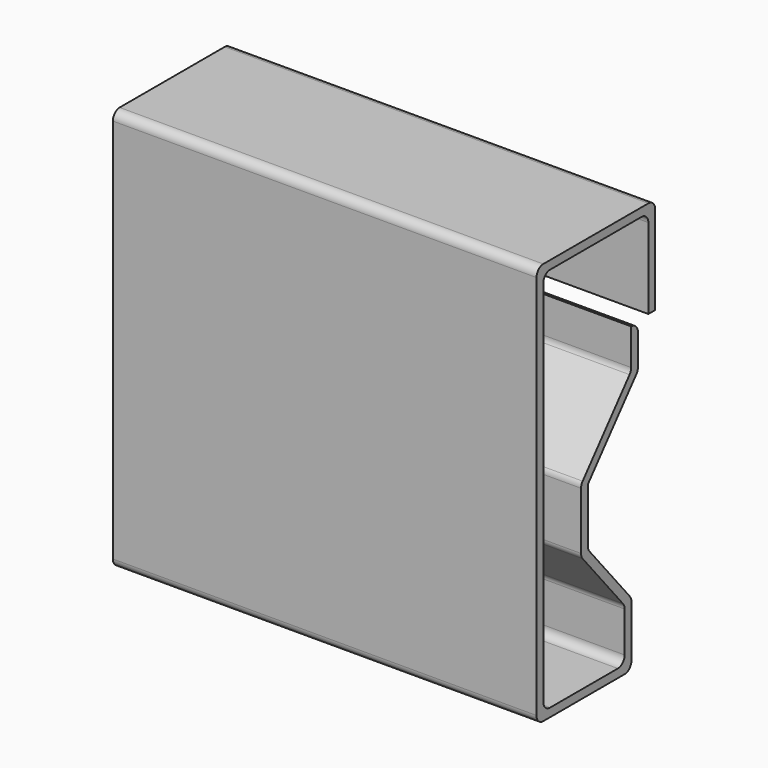
from build123d import *

# Parameters (mm, degrees)
F1_DEPTH = 100
F2_R     = 1.99999


# Not quite as in the source:
# - a fillet or chamfer is up to 0.001 mm smaller than in the source, because OpenCascade refuses the exact size


with BuildPart() as f1:
    # F0 (on Right) → F1 (new body)
    with BuildSketch(Plane.YZ):
        Polygon((33, -23), (35, -23), (35, 0), (0, 0), (0, -95), (28, -95), (28, -80), (15.1442478063, -64.6791111376), (15.1442478063, -51.1349920747), (29.9283628291, -33.5159698829), (29.9283628291, -23.5159698829), (27.9283628291, -23.5159698829), (27.9283628291, -32.7880294144), (13.1442478063, -50.4070516062), (13.1442478063, -65.4070516062), (26, -80.7279404685), (26, -93), (2, -93), (2, -2), (33, -2), align=None)
    extrude(amount=F1_DEPTH)

    # F2 (radius 2 in the source; OpenCascade refuses exactly that, so slightly less here)
    f2_edges = [f1.edges().sort_by_distance(p)[0] for p in [
        (50, 35, 0),
        (50, 0, 0),
        (50, 33, -2),
        (50, 2, -2),
        (50, 0, -95),
        (50, 28, -95),
        (50, 28, -80),
        (50, 2, -93),
        (50, 26, -93),
        (50, 26, -80.72794),
        (50, 27.928363, -32.788029),
        (50, 15.144248, -64.679111),
        (50, 29.928363, -33.51597),
        (50, 29.928363, -23.51597),
        (50, 13.144248, -50.407052),
        (50, 13.144248, -65.407052),
    ]]
    fillet(f2_edges, radius=F2_R)


solid = f1.part
